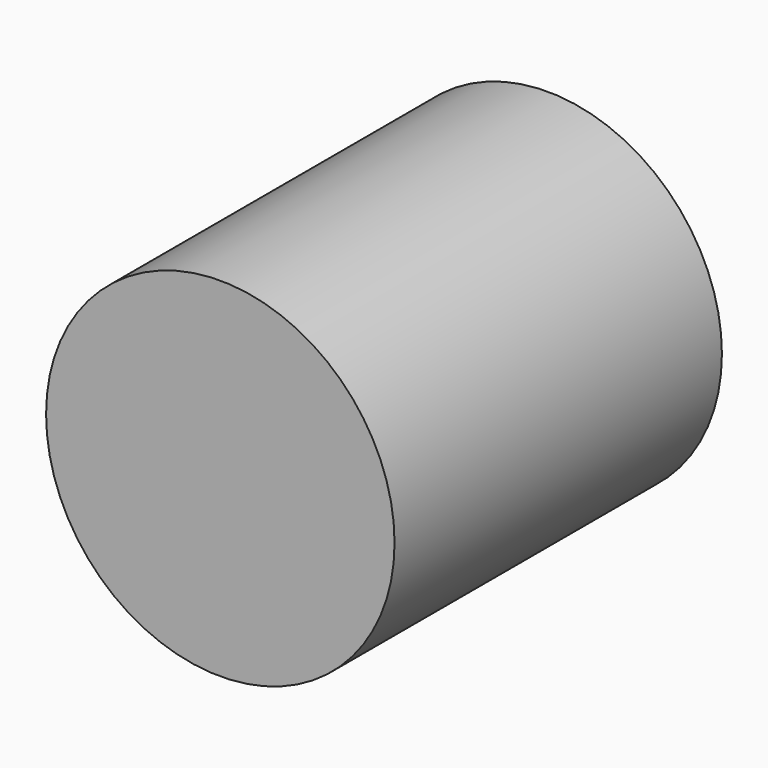
from build123d import *

# Parameters (mm, degrees)
F0_W     = 25.7850475609
F0_H     = 69.0255090594
F1_DEPTH = 97.1566960216
F2_W     = 29.3421596289
F2_H     = 68.0039366707
F3_DEPTH = 74.8365670443
F5_W     = 27.3843407631
F5_H     = 64.3117055297


with BuildPart() as f1:
    # F0 (on Top) → F1 (new body)
    with BuildSketch(Plane.XY):
        with Locations((44.0845470876, 10.3604607284)):
            Rectangle(F0_W, F0_H)
    extrude(amount=F1_DEPTH)

    # F2 (on face) → F3 (join)
    with BuildSketch(Plane.YZ.offset(56.977070868)):
        with Locations((14.6710798144, 47.3301787861)):
            Rectangle(F2_W, F2_H)
    extrude(amount=-F3_DEPTH)


with BuildPart() as f6:
    # F5 (on Top) → F6 (revolve)
    with BuildSketch(Plane.XY):
        with Locations((-27.3843705654, 0.8298419416)):
            Rectangle(F5_W, F5_H)
    revolve(axis=Axis((-13.6922001839, 0.8298419416, 0), (0, -1, 0)))


solid = f6.part
